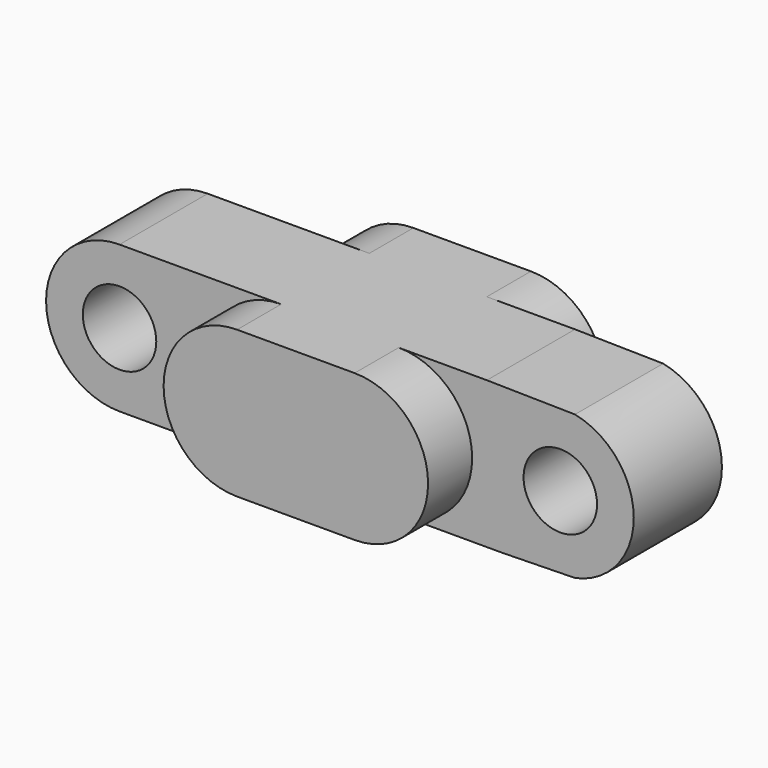
from build123d import *

# Parameters (mm, degrees)
F0_R          = 0.5
F1_DEPTH      = 1.5
F2_DEPTH      = 0.75
F2_DEPTH_BACK = 2.25


# Not quite as in the source:
# - a feature names something its author has since deleted; it is built from what else it names


with BuildPart() as f1:
    # F0 (on Front) → F1 (new body)
    with BuildSketch(Plane.XZ):
        with BuildLine():
            ThreePointArc((-2.4, -2.24940907), (-1.4, -1.24940907), (-2.4, -0.24940907))
            Line((-2.4, -0.24940907), (-4, -0.24940907))
            ThreePointArc((-4, -0.24940907), (-5, -1.24940907), (-4, -2.24940907))
            Line((-4, -2.24940907), (-2.4, -2.24940907))
        make_face()
        with BuildLine():
            Line((0, -0.2696131729), (-1.2, -0.24940907))
            Line((-1.2, -0.24940907), (-2.4, -0.24940907))
            ThreePointArc((-2.4, -0.24940907), (-1.4, -1.24940907), (-2.4, -2.24940907))
            Line((-2.4, -2.24940907), (-1, -2.24940907))
            Line((-1, -2.24940907), (0, -2.2292049671))
            ThreePointArc((0, -2.2292049671), (0.8, -1.24940907), (0, -0.2696131729))
        make_face()
        with Locations((-0.2, -1.24940907)):
            Circle(F0_R, mode=Mode.SUBTRACT)
        with BuildLine():
            ThreePointArc((-4, -2.24940907), (-5, -1.24940907), (-4, -0.24940907))
            Line((-4, -0.24940907), (-6.2, -0.24940907))
            ThreePointArc((-6.2, -0.24940907), (-7.2, -1.24940907), (-6.2, -2.24940907))
            Line((-6.2, -2.24940907), (-4, -2.24940907))
        make_face()
        with Locations((-6.2, -1.24940907)):
            Circle(F0_R, mode=Mode.SUBTRACT)
    extrude(amount=F1_DEPTH)

    # F0 (on Front) → F2 (join, two sides)
    with BuildSketch(Plane.XZ) as f2_sk:
        with BuildLine():
            ThreePointArc((-2.4, -2.24940907), (-1.4, -1.24940907), (-2.4, -0.24940907))
            Line((-2.4, -0.24940907), (-4, -0.24940907))
            ThreePointArc((-4, -0.24940907), (-5, -1.24940907), (-4, -2.24940907))
            Line((-4, -2.24940907), (-2.4, -2.24940907))
        make_face()
    extrude(amount=-F2_DEPTH)
    extrude(f2_sk.sketch, amount=F2_DEPTH_BACK)


solid = f1.part
